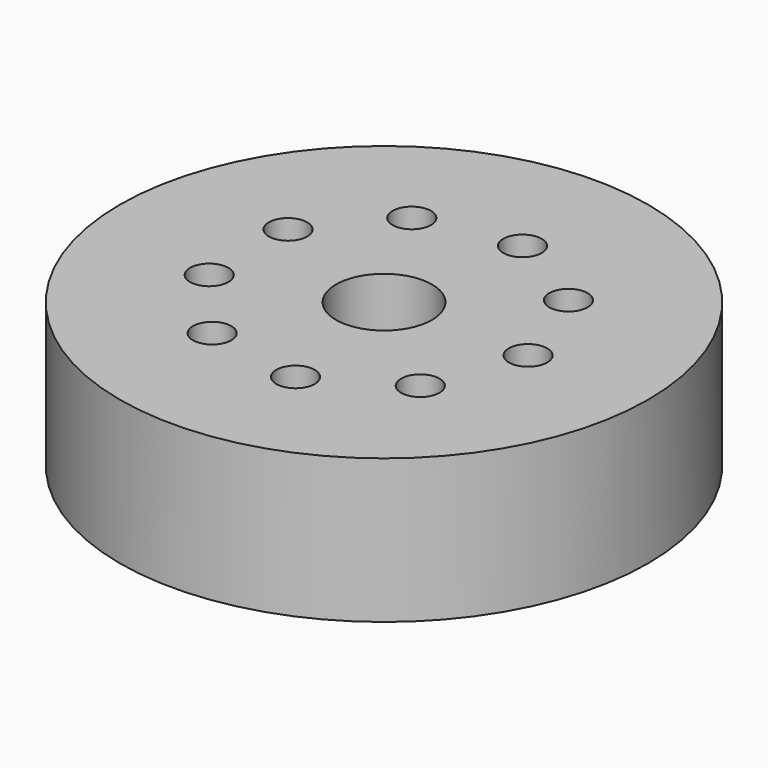
from build123d import *

# Parameters (mm, degrees)
F0_R            = 27.5
F0_R_2          = 5
F1_DEPTH        = 15
F2_R            = 2
F3_DEPTH        = 15.001
F3_COPIES_COUNT = 9


# Not quite as in the source:
# - a pattern or mirror of a feature is missing from the dataset's text; its kind, count and spacing are read off the source's solid


with BuildPart() as f1:
    # F0 (on Top) → F1 (new body)
    with BuildSketch(Plane.XY):
        Circle(F0_R)
        Circle(F0_R_2, mode=Mode.SUBTRACT)
    extrude(amount=F1_DEPTH)

    # F2 (on face) → F3 (cut, through all)
    with BuildSketch(Plane.XY.offset(15)):
        with Locations((15, 0)):
            Circle(F2_R)
    f3 = extrude(amount=-F3_DEPTH, mode=Mode.SUBTRACT)

    # F3_copies: F3 ×9 about axis
    f3_copies_axis = Axis((0, 0, 0), (0, 0, 1))
    for i in range(1, F3_COPIES_COUNT):
        add(f3.rotate(f3_copies_axis, i * 360 / F3_COPIES_COUNT), mode=Mode.SUBTRACT)


solid = f1.part
